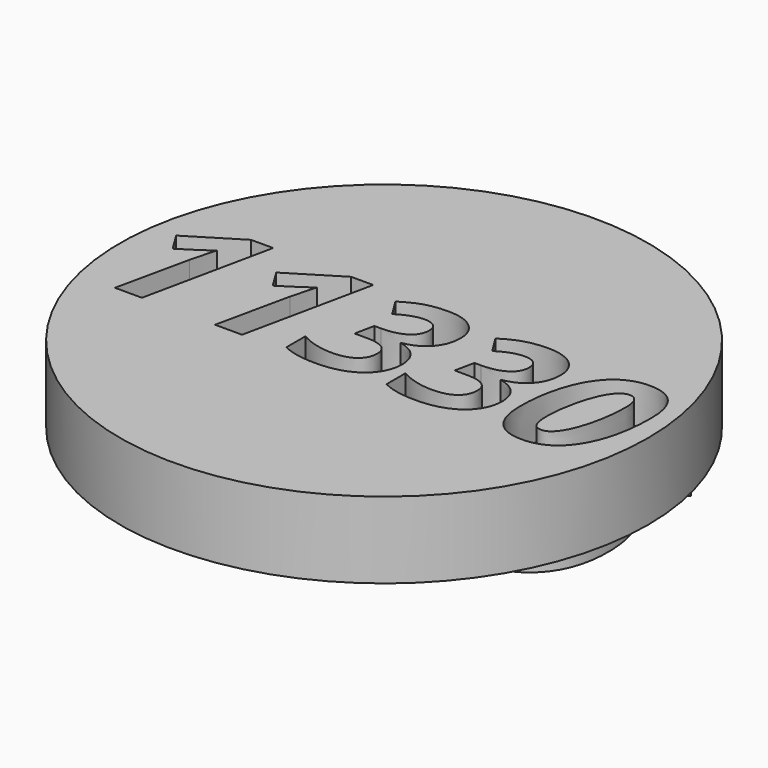
from build123d import *

# Parameters (mm, degrees)
F0_R         = 51.7430433388
F1_DEPTH     = 14.986
F2_TEXT_SIZE = 35.6145228984
F3_DEPTH     = 7.62
F4_TEXT_SIZE = 42.3982403138
F5_DEPTH     = 7.366


# Not quite as in the source:
# - Text() gives the source's letters only with a copy of the font that has no kerning and outlines rounded to 1/6400 em; it was checked with that copy


with BuildPart() as f1:
    # F0 (on Top) → F1 (new body)
    with BuildSketch(Plane.XY):
        Circle(F0_R)
    extrude(amount=F1_DEPTH)

    # F2 (on face) → F3 (cut)
    with BuildSketch(Plane.XY.offset(14.986)):
        with Locations((-49.7632505275, -12.078424282)):
            Text('11330', F2_TEXT_SIZE, font='Open Sans', font_style=FontStyle.BOLDITALIC, text_align=(TextAlign.LEFT, TextAlign.BOTTOM))
    extrude(amount=-F3_DEPTH, mode=Mode.SUBTRACT)


with BuildPart() as f5:
    # F4 (on face) → F5 (new body)
    with BuildSketch(Plane(origin=(0, 0, 0), x_dir=(1, 0, 0), z_dir=(0, 0, -1))):
        with Locations((-46.5155069317, -15.4160009697)):
            Text('QAQ', F4_TEXT_SIZE, font='Open Sans', text_align=(TextAlign.LEFT, TextAlign.BOTTOM))
    extrude(amount=F5_DEPTH)


solid = Compound([f1.part, f5.part])
